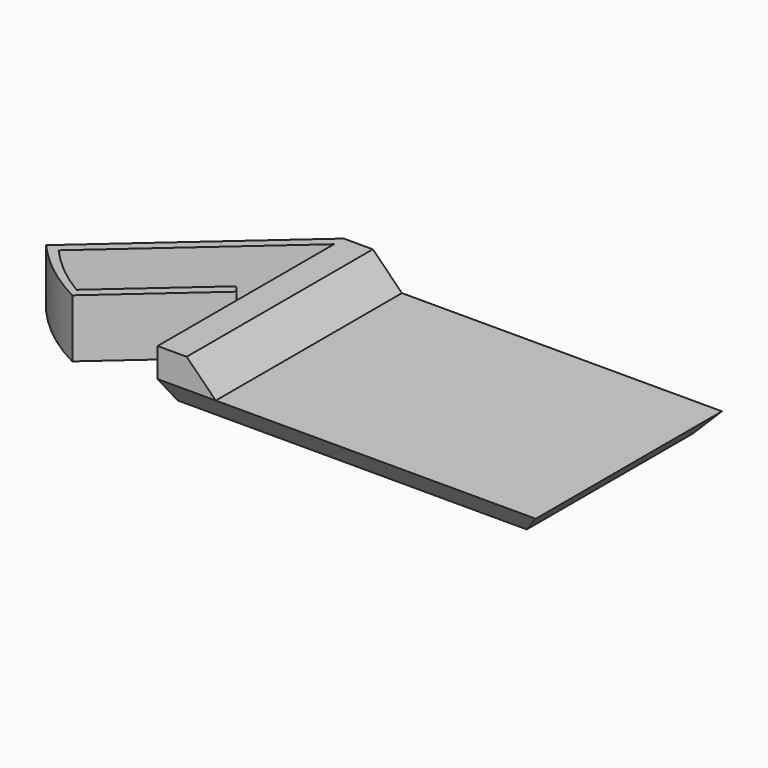
from build123d import *

# Parameters (mm, degrees)
F0_W        = 28.575
F0_H        = 25.4
F1_DEPTH    = 3.175
F2_DEPTH    = 6.35
F3_T4_DEPTH = 58.0603739472
F6_DEPTH    = 25.4
F7_DEPTH    = 50.8


# Not quite as in the source:
# - a fillet or chamfer that OpenCascade refuses, or shapes differently, is made with other operations: its cross-section is extruded or revolved along the edge and cut away or added
# - a feature names something its author has since deleted; it is built from what else it names


with BuildPart() as f1:
    # F0 (on Top) → F1 (new body)
    with BuildSketch(Plane.XY):
        with Locations((14.2875, 0)):
            Rectangle(F0_W, F0_H)
        with BuildLine():
            Line((-9.525, -12.7), (0, -12.7))
            Line((0, -12.7), (0, 12.7))
            Line((0, 12.7), (-9.525, 12.7))
            Line((-9.525, 12.7), (-28.575, -4.1005208253))
            ThreePointArc((-28.575, -4.1005208253), (-25.0870430294, -7.374431916), (-21.0470880315, -9.9362869613))
            Line((-21.0470880315, -9.9362869613), (-10.525, -0.6566775598))
            Line((-10.525, -0.6566775598), (-11.1864378278, 0.0933224402))
            Line((-11.1864378278, 0.0933224402), (-21.3967655869, -8.9113402448))
            ThreePointArc((-21.3967655869, -8.9113402448), (-24.4613665471, -6.7728299311), (-27.1481868608, -4.1755232473))
            Line((-27.1481868608, -4.1755232473), (-9.525, 11.3666666667))
            Line((-9.525, 11.3666666667), (-9.525, -12.7))
        make_face()
    extrude(amount=F1_DEPTH)

    # F0 (on Top) → F2 (join)
    with BuildSketch(Plane.XY):
        with BuildLine():
            Line((-9.525, -12.7), (0, -12.7))
            Line((0, -12.7), (0, 12.7))
            Line((0, 12.7), (-9.525, 12.7))
            Line((-9.525, 12.7), (-28.575, -4.1005208253))
            ThreePointArc((-28.575, -4.1005208253), (-25.0870430294, -7.374431916), (-21.0470880315, -9.9362869613))
            Line((-21.0470880315, -9.9362869613), (-10.525, -0.6566775598))
            Line((-10.525, -0.6566775598), (-11.1864378278, 0.0933224402))
            Line((-11.1864378278, 0.0933224402), (-21.3967655869, -8.9113402448))
            ThreePointArc((-21.3967655869, -8.9113402448), (-24.4613665471, -6.7728299311), (-27.1481868608, -4.1755232473))
            Line((-27.1481868608, -4.1755232473), (-9.525, 11.3666666667))
            Line((-9.525, 11.3666666667), (-9.525, -12.7))
        make_face()
    extrude(amount=F2_DEPTH)

    # F3: chamfer of 6.35 on 1 edges, made by hand


with BuildPart() as f3_tool2:
    # F3_s3 → F3_t4 (new body)
    with BuildSketch(Plane.XZ.offset(29.0301869736)):
        Polygon((0, 0), (-6.35, 6.35), (0, 6.35), align=None)
    extrude(amount=-F3_T4_DEPTH)

    split(bisect_by=Plane.XY.offset(3.175), keep=Keep.TOP)


with BuildPart() as f1_1:
    add(f1.part)

    # F3_t1: cut F3_tool2
    add(f3_tool2.part, mode=Mode.SUBTRACT)

    # F5 (on face) → F6 (join)
    with BuildSketch(Plane(origin=(0, 12.7, 0), x_dir=(-1, 0, 0), z_dir=(0, 1, 0))):
        Polygon((3.175, 3.175), (-28.575, 3.175), (-28.575, 0), (9.525, 0), (9.525, 6.35), (6.35, 6.35), align=None)
        Polygon((-28.575, 0), (-28.575, 3.175), (-31.75, 3.175), align=None)
    extrude(amount=-F6_DEPTH)

    # F4 (on face) → F7 (cut)
    with BuildSketch(Plane(origin=(-9.525, 0, 0), x_dir=(0, -1, 0), z_dir=(-1, 0, 0))):
        Polygon((9.9561735988, 0), (12.7, 0), (12.7, 3.175), align=None)
    extrude(amount=-F7_DEPTH, mode=Mode.SUBTRACT)


solid = f1_1.part
